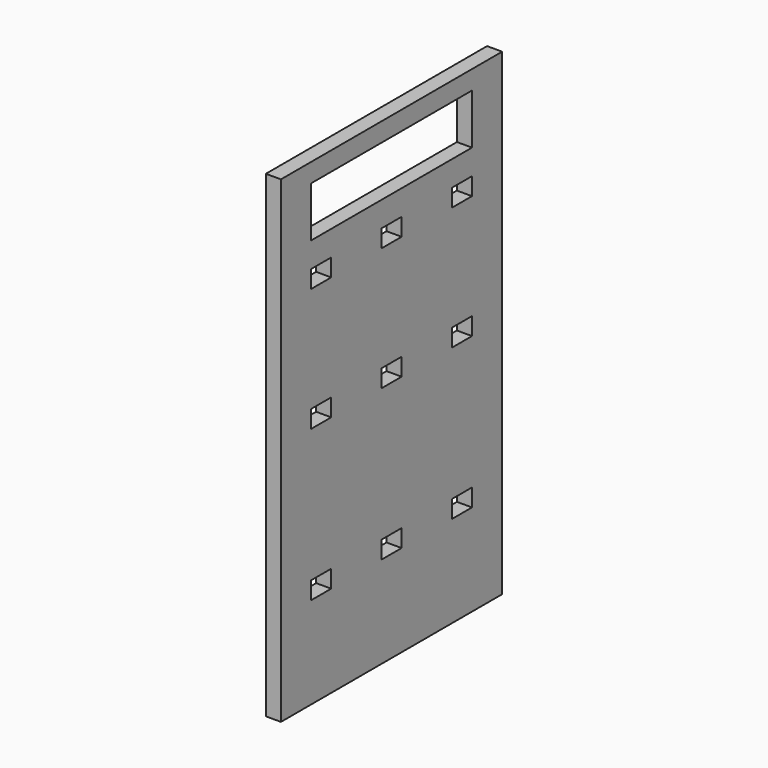
from build123d import *

# Parameters (mm, degrees)
F1_DEPTH = 6


with BuildPart() as f1:
    # F0 (on Right) → F1 (new body)
    with BuildSketch(Plane.YZ):
        Polygon((62.5, 142.2184194922), (9.4337919727, 142.2184194922), (9.4337919727, 134.7184194922), (47.5, 134.7184194922), (47.5, 129.8368871212), (62.5, 129.8368871212), align=None)
        Polygon((9.4337919727, 142.2184194922), (-47.5, 142.2184194922), (-47.5, -47.7815805078), (62.5, -47.7815805078), (62.5, 129.8368871212), (47.5, 129.8368871212), (47.5, 114.7184194922), (-32.5, 114.7184194922), (-32.5, 134.7184194922), (9.4337919727, 134.7184194922), align=None)
        Polygon((-22.5, -4.2815805078), (-22.5, -7.7815805078), (-22.5, -11.2815805078), (-32.5, -11.2815805078), (-32.5, -4.2815805078), align=None, mode=Mode.SUBTRACT)
        Polygon((12.5, -4.2815805078), (12.5, -7.7815805078), (12.5, -11.2815805078), (2.5, -11.2815805078), (2.5, -7.7815805078), (2.5, -4.2815805078), align=None, mode=Mode.SUBTRACT)
        Polygon((37.5, -7.7815805078), (37.5, -4.2815805078), (47.5, -4.2815805078), (47.5, -11.2815805078), (37.5, -11.2815805078), align=None, mode=Mode.SUBTRACT)
        Polygon((-22.5, 55.7184194922), (-22.5, 52.2184194922), (-22.5, 48.7184194922), (-32.5, 48.7184194922), (-32.5, 55.7184194922), align=None, mode=Mode.SUBTRACT)
        Polygon((-22.5, 101.2184194922), (-22.5, 97.7184194922), (-32.5, 97.7184194922), (-32.5, 104.7184194922), (-22.5, 104.7184194922), align=None, mode=Mode.SUBTRACT)
        Polygon((12.5, 55.7184194922), (12.5, 52.2184194922), (12.5, 48.7184194922), (2.5, 48.7184194922), (2.5, 52.2184194922), (2.5, 55.7184194922), align=None, mode=Mode.SUBTRACT)
        Polygon((37.5, 52.2184194922), (37.5, 55.7184194922), (47.5, 55.7184194922), (47.5, 48.7184194922), (37.5, 48.7184194922), align=None, mode=Mode.SUBTRACT)
        Polygon((2.5, 97.7184194922), (2.5, 101.2184194922), (2.5, 104.7184194922), (12.5, 104.7184194922), (12.5, 101.2184194922), (12.5, 97.7184194922), align=None, mode=Mode.SUBTRACT)
        Polygon((37.5, 97.7184194922), (37.5, 101.2184194922), (37.5, 104.7184194922), (47.5, 104.7184194922), (47.5, 97.7184194922), align=None, mode=Mode.SUBTRACT)
    extrude(amount=F1_DEPTH)


solid = f1.part
